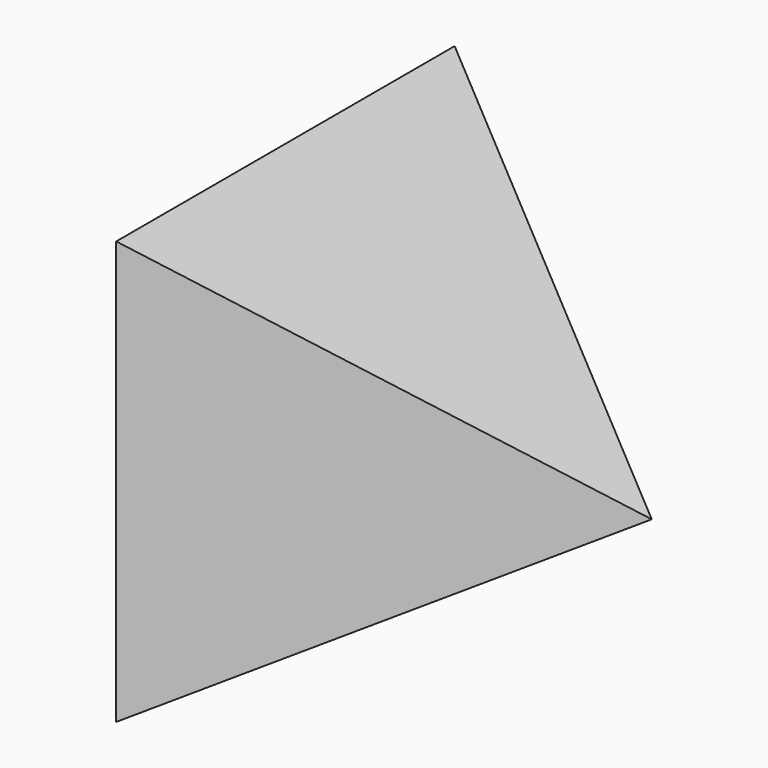
from build123d import *

# Parameters (mm, degrees)
F0_W = 76.2
F0_H = 76.2


# Not quite as in the source:
# - an extrude whose draft closes it to a point is written as a loft to that point


with BuildPart() as f1:
    # F0 (on Right) → F1 section 0
    with BuildSketch(Plane.YZ, mode=Mode.PRIVATE) as f1_s0:
        with Locations((44.4602915034, 23.4026159108)):
            Rectangle(F0_W, F0_H)
    loft([f1_s0.sketch, Vertex(65.9911357684, 44.4602915034, 23.4026159108)], ruled=True)


solid = f1.part
